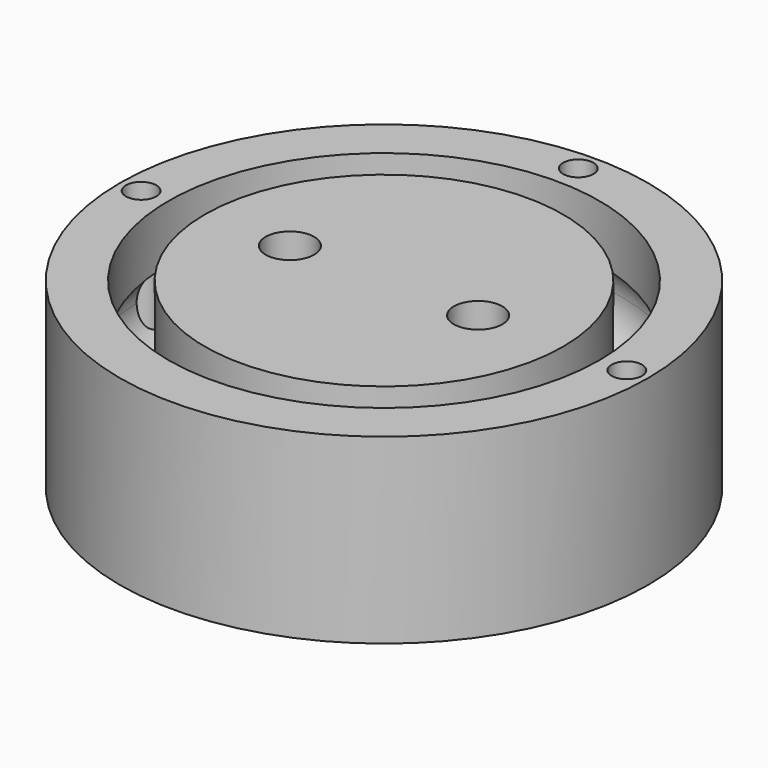
from build123d import *

# Parameters (mm, degrees)
F0_R      = 21.75
F0_R_2    = 17.75
F1_DEPTH  = 15
F0_R_3    = 14.75
F0_R_4    = 4
F9_DEPTH  = 7
F11_D     = 4
F10_R     = 3.75
F12_DEPTH = 10
F14_D     = 2.5
F16_DEPTH = 2
F17_DEPTH = 4.5


with BuildPart() as f1:
    # F0 (on Top) → F1 (new body)
    with BuildSketch(Plane.XY):
        Circle(F0_R)
        Circle(F0_R_2, mode=Mode.SUBTRACT)
    extrude(amount=-F1_DEPTH)


with BuildPart() as f1b:
    # F0 (on Top) → F1, piece 2 (new body)
    with BuildSketch(Plane.XY):
        Circle(F0_R_3)
        Circle(F0_R_4, mode=Mode.SUBTRACT)
        Circle(F0_R_4)
    extrude(amount=-F1_DEPTH)


with BuildPart() as f6_tool:
    # F4 (on Right) → F6 (revolve)
    with BuildSketch(Plane.YZ):
        with BuildLine():
            Line((17.75, -10.3831406487), (17.75, -4.6168593513))
            ThreePointArc((17.75, -4.6168593513), (13, -7.5), (17.75, -10.3831406487))
        make_face()
        with BuildLine():
            ThreePointArc((17.75, -10.3831406487), (19.0282638464, -9.1863421954), (19.5, -7.5))
            ThreePointArc((19.5, -7.5), (19.0282638464, -5.8136578046), (17.75, -4.6168593513))
            Line((17.75, -4.6168593513), (17.75, -10.3831406487))
        make_face()
    revolve(axis=Axis((0, 0, 0), (0, 0, 1)))


with BuildPart() as f1_1:
    add(f1.part)

    # F6: cut by f6_tool
    add(f6_tool.part, mode=Mode.SUBTRACT)


with BuildPart() as f1b_1:
    add(f1b.part)

    # F6: cut by f6_tool
    add(f6_tool.part, mode=Mode.SUBTRACT)


with BuildPart() as f9_tool:
    # F8 (on face) → F9 (new body)
    with BuildSketch(Plane(origin=(0, 0, -15), x_dir=(1, 0, 0), z_dir=(0, 0, -1))):
        with BuildLine():
            ThreePointArc((-3.1796149168, 17.462890625), (0, 17.75), (3.1796149168, 17.462890625))
            ThreePointArc((3.1796149168, 17.462890625), (0, 19.5), (-3.1796149168, 17.462890625))
        make_face()
        with BuildLine():
            ThreePointArc((-3.1796149168, 17.462890625), (-0.7487816074, 12.5810343517), (3.5, 16))
            ThreePointArc((3.5, 16), (3.4189656483, 16.7487816074), (3.1796149168, 17.462890625))
            ThreePointArc((3.1796149168, 17.462890625), (0, 17.75), (-3.1796149168, 17.462890625))
        make_face()
    extrude(amount=-F9_DEPTH)


with BuildPart() as f1_2:
    add(f1_1.part)

    # F9: cut by f9_tool
    add(f9_tool.part, mode=Mode.SUBTRACT)

    # F14 (through all)
    with Locations(Plane(origin=(0, 0, -15), x_dir=(1, 0, 0), z_dir=(0, 0, -1))):
        with Locations((-20, 0), (0, -20), (20, 0)):
            Hole(F14_D / 2)


with BuildPart() as f1b_2:
    add(f1b_1.part)

    # F9: cut by f9_tool
    add(f9_tool.part, mode=Mode.SUBTRACT)

    # F11 (through all)
    with Locations(Plane(origin=(0, 0, -15), x_dir=(1, 0, 0), z_dir=(0, 0, -1))):
        with Locations((-7.75, 0), (7.75, 0)):
            Hole(F11_D / 2)

    # F10 (on face) → F12 (cut)
    with BuildSketch(Plane(origin=(0, 0, -15), x_dir=(1, 0, 0), z_dir=(0, 0, -1))):
        with Locations((-7.75, 0)):
            Circle(F10_R)
        with Locations((7.75, 0)):
            Circle(F10_R)
    extrude(amount=-F12_DEPTH, mode=Mode.SUBTRACT)


with BuildPart() as f16:
    # F15 (on face) → F16 (new body)
    with BuildSketch(Plane(origin=(0, 0, -15), x_dir=(1, 0, 0), z_dir=(0, 0, -1))):
        with BuildLine():
            ThreePointArc((-3.1210564717, 14.416015625), (0, 12.5), (3.1210564717, 14.416015625))
            ThreePointArc((3.1210564717, 14.416015625), (0, 14.75), (-3.1210564717, 14.416015625))
        make_face()
        with BuildLine():
            ThreePointArc((-5.0425818511, 13.8612722459), (0, 10.5), (5.0425818511, 13.8612722459))
            ThreePointArc((5.0425818511, 13.8612722459), (4.0912324207, 14.1712496725), (3.1210564717, 14.416015625))
            ThreePointArc((3.1210564717, 14.416015625), (0, 12.5), (-3.1210564717, 14.416015625))
            ThreePointArc((-3.1210564717, 14.416015625), (-4.0912324207, 14.1712496725), (-5.0425818511, 13.8612722459))
        make_face()
    extrude(amount=F16_DEPTH)

    # F15 (on face) → F17 (join)
    with BuildSketch(Plane(origin=(0, 0, -15), x_dir=(1, 0, 0), z_dir=(0, 0, -1))):
        with BuildLine():
            ThreePointArc((-3.1210564717, 14.416015625), (0, 12.5), (3.1210564717, 14.416015625))
            ThreePointArc((3.1210564717, 14.416015625), (0, 14.75), (-3.1210564717, 14.416015625))
        make_face()
    extrude(amount=-F17_DEPTH)


solid = Compound([f1_2.part, f1b_2.part, f16.part])
